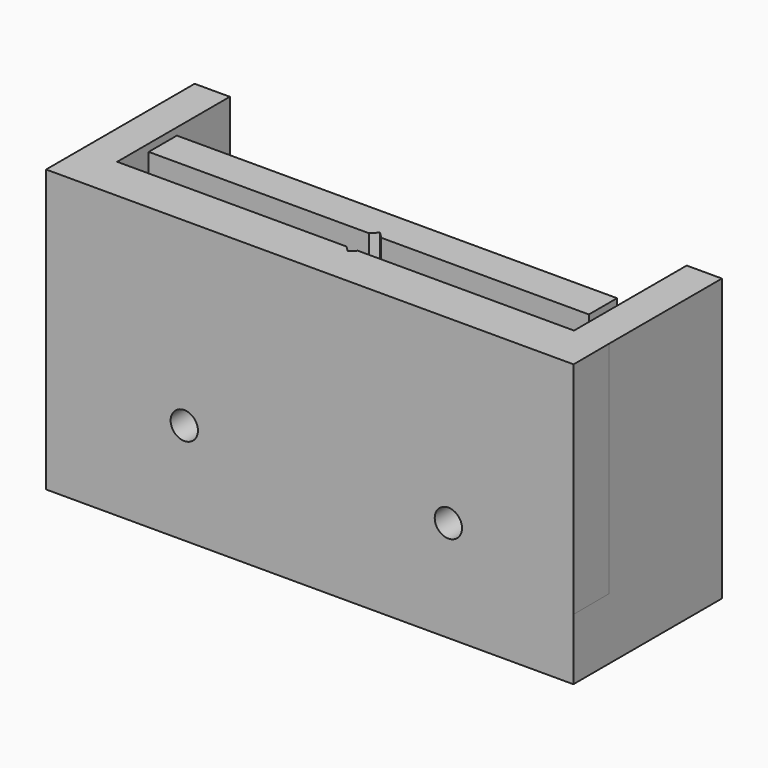
from build123d import *

# Parameters (mm, degrees)
F1_DEPTH = 25
F2_R     = 1.55
F3_DEPTH = 2
F4_DEPTH = 25
F6_DEPTH = 7
F7_DEPTH = 12


with BuildPart() as f1:
    # F0 (on Top) → F1 (new body)
    with BuildSketch(Plane.XY):
        Polygon((0, -3.165672766), (-0.6428928915, -2.5227798745), (-26.700000003, -2.5227798615), (-26.700000003, 13.4772201385), (-30.700000003, 13.4772201385), (-30.700000003, -2.5227798615), (-30.700000003, -7.615136914), (29.2246248573, -7.615136914), (29.2000018954, -2.5227798615), (29.2000018954, 13.4772201385), (25.2000018954, 13.4772201385), (25.2000018954, -2.5227798615), (23, -2.5227798745), (0.6428928915, -2.5227798745), align=None)
    extrude(amount=F1_DEPTH)


with BuildPart() as f1b:
    # F0 (on Top) → F1, piece 2 (new body)
    with BuildSketch(Plane.XY):
        Polygon((-0.7071006365, 0.7182756418), (0, 1.4253762783), (0.7071067812, 0.7182694971), (0.7043308199, 0.7154935358), (24.2928932188, 0.7182694971), (24.2928932188, 4.7182694971), (-25.7071067812, 4.7182694971), (-25.7071067812, 0.7123853715), (-0.7041527766, 0.715327782), align=None)
    extrude(amount=F1_DEPTH)

    # F2 (on face) → F3 (cut)
    with BuildSketch(Plane(origin=(0, 4.7182694971, 0), x_dir=(-1, 0, 0), z_dir=(0, 1, 0))):
        Polygon((-11.9, 2.7102141655), (-11.9, 6.2897858345), (-15, 8.079571669), (-18.1, 6.2897858345), (-18.1, 2.7102141655), (-15, 0.920428331), align=None)
        with Locations((-15, 4.5)):
            Circle(F2_R, mode=Mode.SUBTRACT)
        Polygon((11.9, 6.2897858345), (11.9, 2.7102141655), (15, 0.920428331), (18.1, 2.7102141655), (18.1, 6.2897858345), (15, 8.079571669), align=None)
        with Locations((15, 4.5)):
            Circle(F2_R, mode=Mode.SUBTRACT)
    extrude(amount=-F3_DEPTH, mode=Mode.SUBTRACT)


with BuildPart() as f4_tool:
    # F4 (cut): faces of the model
    f4_faces = [f1b.part.faces().sort_by_distance(p)[0] for p in [
        (-15, 4.7182694971, 4.5),
        (15, 4.7182694971, 4.5),
    ]]
    extrude(f4_faces, amount=-F4_DEPTH)


with BuildPart() as f1_1:
    add(f1.part)

    # F4: cut by f4_tool
    add(f4_tool.part, mode=Mode.SUBTRACT)

    # F5 (on face) → F6 (join)
    with BuildSketch(Plane(origin=(0, 0, 0), x_dir=(1, 0, 0), z_dir=(0, 0, -1))):
        with BuildLine():
            Line((-3.1019229725, -2.1028676977), (-30.700000003, 7.615136914))
            Line((-30.700000003, 7.615136914), (-30.700000003, -13.4772201385))
            Line((-30.700000003, -13.4772201385), (-3.1020298452, -3.7632462614))
            ThreePointArc((-3.1020298452, -3.7632462614), (-3.2438445731, -2.933047848), (-3.1019229725, -2.1028676977))
        make_face()
        with BuildLine():
            Line((29.2000018954, 7.615136914), (-30.700000003, 7.615136914))
            Line((-30.700000003, 7.615136914), (-3.1019229725, -2.1028676977))
            ThreePointArc((-3.1019229725, -2.1028676977), (-0.7436836622, -0.4332087692), (1.6143406887, -2.1031712668))
            Line((1.6143406887, -2.1031712668), (29.2000018954, 7.6064700878))
            Line((29.2000018954, 7.6064700878), (29.2000018954, 7.615136914))
        make_face()
        with BuildLine():
            Line((-3.1020298452, -3.7632462614), (-30.700000003, -13.4772201385))
            Line((-30.700000003, -13.4772201385), (29.2000018954, -13.4772201385))
            Line((29.2000018954, -13.4772201385), (1.614233816, -3.7635498304))
            ThreePointArc((1.614233816, -3.7635498304), (-0.7440054943, -5.4332087589), (-3.1020298452, -3.7632462614))
        make_face()
        with BuildLine():
            Line((29.2000018954, -13.4772201385), (29.2000018954, 7.6064700878))
            Line((29.2000018954, 7.6064700878), (1.6143406887, -2.1031712668))
            ThreePointArc((1.6143406887, -2.1031712668), (1.7204467161, -2.5121762043), (1.7561554217, -2.9332087641))
            ThreePointArc((1.7561554217, -2.9332087641), (1.7204196107, -3.3543999405), (1.614233816, -3.7635498304))
            Line((1.614233816, -3.7635498304), (29.2000018954, -13.4772201385))
        make_face()
    extrude(amount=F6_DEPTH)

    # F0 (on Top) → F7, piece 2 (join)
    with BuildSketch(Plane.XY):
        Polygon((0.6428928915, -2.5227798745), (-0.6428928915, -2.5227798745), (0, -3.165672766), align=None)
    extrude(amount=F7_DEPTH)


with BuildPart() as f1b_1:
    add(f1b.part)

    # F4: cut by f4_tool
    add(f4_tool.part, mode=Mode.SUBTRACT)

    # F0 (on Top) → F7 (join)
    with BuildSketch(Plane.XY):
        Polygon((0.7071067812, 0.7182694971), (0, 1.4253762783), (-0.7071006365, 0.7182756418), (-0.7041527766, 0.715327782), align=None)
    extrude(amount=F7_DEPTH)


solid = Compound([f1_1.part, f1b_1.part])
